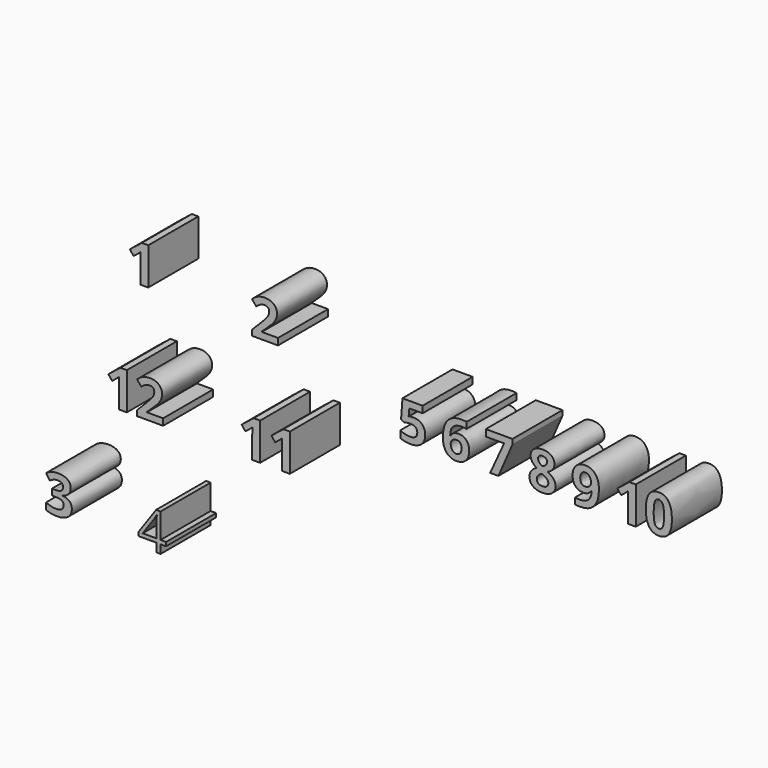
from build123d import *

# Parameters (mm, degrees)
F0_TEXT_SIZE = 10.5833333333
F1_DEPTH     = 12.7


# Not quite as in the source:
# - Text() gives the source's letters only with a copy of the font that has no kerning and outlines rounded to 1/6400 em; it was checked with that copy


with BuildPart() as f1:
    # F0 (on Front) → F1 (new body)
    with BuildSketch(Plane.XZ):
        with Locations((-48.2237284357, 46.8085824676)):
            Text('1', F0_TEXT_SIZE, font='Open Sans', font_style=FontStyle.BOLD, text_align=(TextAlign.LEFT, TextAlign.BOTTOM))
        with Locations((-52.5780126447, 23.0777207084)):
            Text('12', F0_TEXT_SIZE, font='Open Sans', font_style=FontStyle.BOLD, text_align=(TextAlign.LEFT, TextAlign.BOTTOM))
        with Locations((-23.2063625008, 45.0272702622)):
            Text('2', F0_TEXT_SIZE, font='Open Sans', font_style=FontStyle.BOLD, text_align=(TextAlign.LEFT, TextAlign.BOTTOM))
        with Locations((-25.51545389, 22.8600011218)):
            Text('11', F0_TEXT_SIZE, font='Open Sans', font_style=FontStyle.BOLD, text_align=(TextAlign.LEFT, TextAlign.BOTTOM))
        with Locations((-65.0009065866, 0)):
            Text('3', F0_TEXT_SIZE, font='Open Sans', font_style=FontStyle.BOLD, text_align=(TextAlign.LEFT, TextAlign.BOTTOM))
        with Locations((-46.0663661361, 0)):
            Text('4', F0_TEXT_SIZE, font='Open Sans', text_align=(TextAlign.LEFT, TextAlign.BOTTOM))
        with Locations((6.8118176423, 36.2527289438)):
            Text('5 6 7 8 9 10', F0_TEXT_SIZE, font='Open Sans', font_style=FontStyle.BOLD, text_align=(TextAlign.LEFT, TextAlign.BOTTOM))
    extrude(amount=F1_DEPTH)


solid = f1.part
